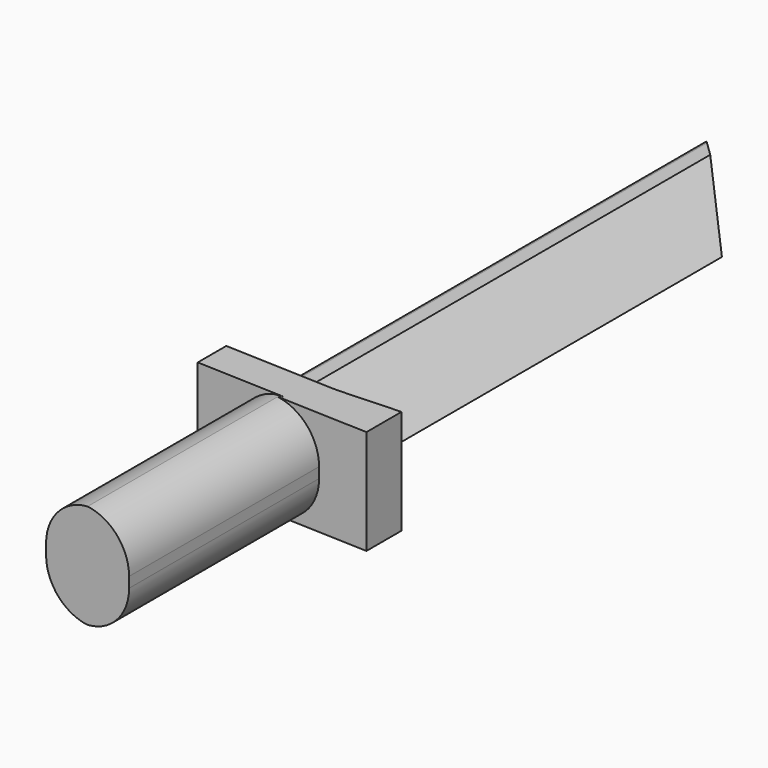
from build123d import *

# Parameters (mm, degrees)
F1_DEPTH      = 3.175
F1_DEPTH_BACK = 3.175
F2_DEPTH      = 6.35
F2_DEPTH_BACK = 6.35
F3_SIZE       = 6.34999
F4_R          = 5.715
F5_R          = 0.635


# Not quite as in the source:
# - a fillet or chamfer is up to 0.001 mm smaller than in the source, because OpenCascade refuses the exact size


with BuildPart() as f1:
    # F0 (on Top) → F1 (new body, two sides)
    with BuildSketch(Plane.XY) as f1_sk:
        Polygon((-41.6700830699, 59.9633481442), (-41.6700830699, -6.6100518558), (-32.9213373307, -6.9480776483), (-32.9213373307, 51.4719223517), align=None)
    extrude(amount=F1_DEPTH)
    extrude(f1_sk.sketch, amount=-F1_DEPTH_BACK)

    # F0 (on Top) → F2 (join, two sides)
    with BuildSketch(Plane.XY) as f2_sk:
        Polygon((-32.9213373307, -6.9480776483), (-41.6700830699, -6.6100518558), (-46.7643177352, -6.4132256179), (-46.7643177352, -10.747612454), (-41.6700830699, -10.9444386919), (-41.6700830699, -40.1244200766), (-31.2753289716, -40.5260427889), (-31.2753289716, -11.7029547691), (-25.3439064165, -11.9321274837), (-25.3439064165, -6.6100518558), align=None)
    extrude(amount=F2_DEPTH)
    extrude(f2_sk.sketch, amount=-F2_DEPTH_BACK)

    # F3 (size 6.35 in the source; OpenCascade refuses exactly that, so slightly less here)
    f3_edges = [f1.edges().sort_by_distance(p)[0] for p in [
        (-32.921337, 22.261922, 3.175),
    ]]
    chamfer(f3_edges, length=F3_SIZE)

    # F4 (call 1 of 4: OpenCascade refuses the feature's edges together)
    f4_edges = [f1.edges().sort_by_distance(p)[0] for p in [
        (-31.275329, -26.114499, 6.35),
    ]]
    fillet(f4_edges, radius=F4_R)

    # F4#2 (call 2 of 4)
    f4_2_edges = [f1.edges().sort_by_distance(p)[0] for p in [
        (-41.670083, -25.534429, 6.35),
    ]]
    fillet(f4_2_edges, radius=F4_R)

    # F4#3 (call 3 of 4)
    f4_3_edges = [f1.edges().sort_by_distance(p)[0] for p in [
        (-31.275329, -26.114499, -6.35),
    ]]
    fillet(f4_3_edges, radius=F4_R)

    # F4#4 (call 4 of 4)
    f4_4_edges = [f1.edges().sort_by_distance(p)[0] for p in [
        (-41.670083, -25.534429, -6.35),
    ]]
    fillet(f4_4_edges, radius=F4_R)

    # F5
    f5_edges = [f1.edges().sort_by_distance(p)[0] for p in [
        (-41.670083, 26.676648, 3.175),
    ]]
    fillet(f5_edges, radius=F5_R)


solid = f1.part
